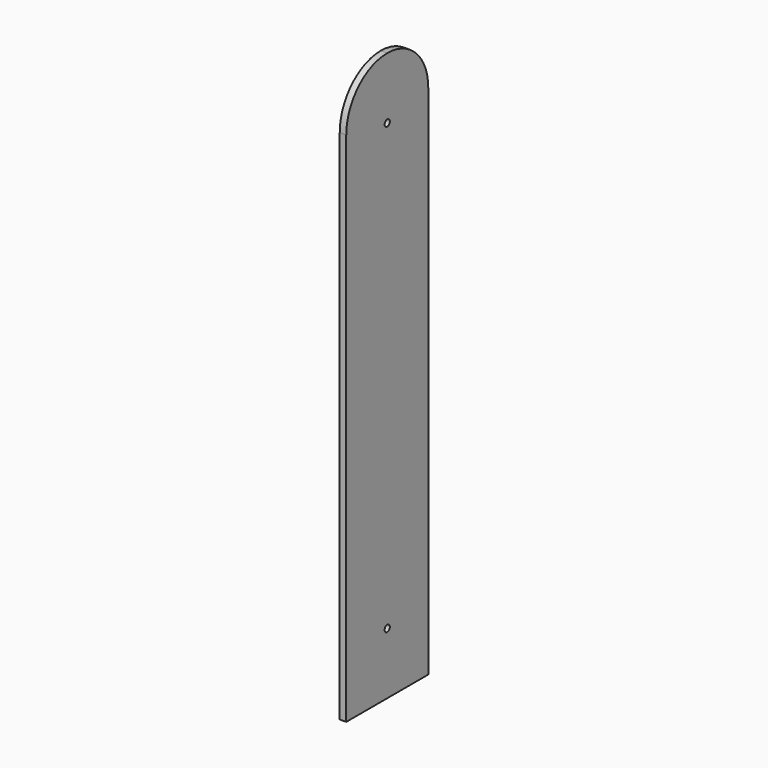
from build123d import *

# Parameters (mm, degrees)
F1_W     = 50
F1_H     = 277
F1_R     = 1.5875
F2_DEPTH = 1.5875
F3_R     = 24.99999


# Not quite as in the source:
# - a fillet or chamfer is up to 0.001 mm smaller than in the source, because OpenCascade refuses the exact size
# - a length typed as a fraction of an inch, garbled in the dataset ("3 / 203.2 mm" for 3/8 in), is restored


with BuildPart() as f2:
    # F1 (on Right) → F2 (new body, symmetric)
    with BuildSketch(Plane.YZ):
        Rectangle(F1_W, F1_H)
        with Locations((0, -108.5)):
            Circle(F1_R, mode=Mode.SUBTRACT)
        with Locations((0, 108.5)):
            Circle(F1_R, mode=Mode.SUBTRACT)
    extrude(amount=F2_DEPTH, both=True)

    # F3 (radius 25 in the source; OpenCascade refuses exactly that, so slightly less here)
    f3_edges = [f2.edges().sort_by_distance(p)[0] for p in [
        (0, -25, 138.5),
        (0, 25, 138.5),
    ]]
    fillet(f3_edges, radius=F3_R)


solid = f2.part
